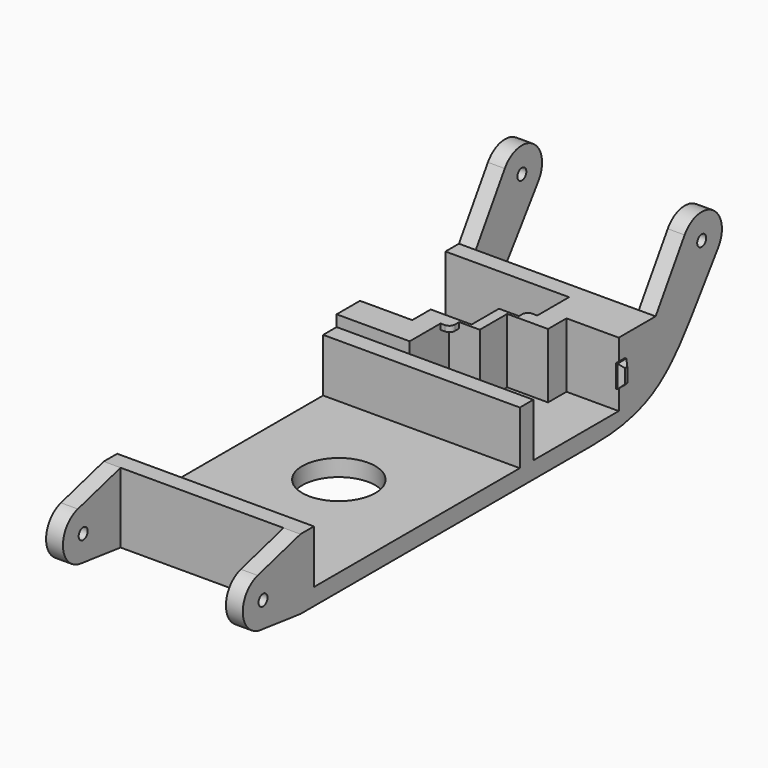
from build123d import *

# Parameters (mm, degrees)
F0_R      = 6.5
F0_W      = 34.999999702
F0_H      = 3
F0_H_2    = 0.3
F1_DEPTH  = 3
F2_DEPTH  = 9.5
F3_DEPTH  = 11.5
F5_DEPTH  = 3
F7_DEPTH  = 3
F8_R      = 1
F9_DEPTH  = 35.000999702
F11_DEPTH = 1
F13_DEPTH = 1
F14_SIZE  = 0.75
F15_W     = 1.8819853365
F15_H     = 1.731043148
F15_W_2   = 1.7636035271
F15_H_2   = 1.938064149
F16_DEPTH = 1
F18_DEPTH = 36.000999702
F19_R     = 1


# Not quite as in the source:
# - ends of sketch curves that miss each other by under 0.0002 mm in the source are joined
# - a feature names something its author has since deleted; it is built from what else it names


with BuildPart() as f1:
    # F0 (on Top) → F1 (new body)
    with BuildSketch(Plane.XY):
        Polygon((7.8607099131, 16.1003852367), (-9.6392899379, 16.1003852367), (-9.6392899379, -29.3996147633), (25.3607097641, -29.3996147633), (25.3607097641, 16.1003852367), align=None)
        with Locations((7.8607099131, -2.2867515218)):
            Circle(F0_R, mode=Mode.SUBTRACT)
        with Locations((7.8607099131, -31.1996147633)):
            Rectangle(F0_W, F0_H)
        Polygon((-9.6392899379, 19.1003852367), (-9.6392899379, 16.1003852367), (7.8607099131, 16.1003852367), (25.3607097641, 16.1003852367), (25.3607097641, 19.1003852367), (22.192974557, 19.1003852367), (3.3607097641, 19.1003852367), align=None)
        Polygon((-9.6392899379, 46.3003852367), (-9.6392899379, 43.3003852367), (-6.4715547308, 43.3003852367), (12.3607100621, 43.3003852367), (25.3607097641, 43.3003852367), (25.3607097641, 46.3003852367), align=None)
        with Locations((7.8607099131, -29.5496147633)):
            Rectangle(F0_W, F0_H_2)
        Polygon((16.0607097641, 38.1003852367), (25.3607097641, 38.1003852367), (25.3607097641, 43.3003852367), (12.3607100621, 43.3003852367), (12.3607100621, 35.3003852367), (12.3607100621, 34.5003852367), (7.8607097641, 34.5003852367), (7.8607100621, 33.9926332235), (8.7954637781, 33.9926332235), (16.0607097641, 33.9926332235), align=None)
        Polygon((-9.6392899379, 24.3003852367), (-9.6392899379, 19.1003852367), (3.3607097641, 19.1003852367), (3.3607097641, 27.1003852367), (3.3607097641, 27.9003852367), (7.8607100621, 27.9003852367), (7.8607100621, 28.4081372499), (6.9259563461, 28.4081372499), (-0.3392899379, 28.4081372499), (-0.3392899379, 24.3003852367), align=None)
        Polygon((6.9259563461, 34.5003852367), (6.9259563461, 28.4081372499), (7.8607097641, 28.4081372499), (7.8607100621, 33.9926332235), (7.8607100621, 34.5003852367), align=None)
        Polygon((7.8607100621, 28.4081372499), (7.8607100621, 27.9003852367), (8.7954637781, 27.9003852367), (8.7954637781, 33.9926332235), (7.8607097641, 33.9926332235), align=None)
        Polygon((-9.6392899379, 43.3003852367), (-9.6392899379, 24.3003852367), (-0.3392899379, 24.3003852367), (-0.3392899379, 28.4081372499), (6.9259563461, 28.4081372499), (6.9259563461, 34.5003852367), (7.8607100621, 34.5003852367), (12.3607100621, 34.5003852367), (12.3607100621, 35.3003852367), (12.3607100621, 43.3003852367), (-6.4715547308, 43.3003852367), align=None)
        Polygon((3.3607097641, 27.1003852367), (3.3607097641, 19.1003852367), (22.192974557, 19.1003852367), (25.3607097641, 19.1003852367), (25.3607097641, 38.1003852367), (16.0607097641, 38.1003852367), (16.0607097641, 33.9926332235), (8.7954637781, 33.9926332235), (8.7954637781, 27.9003852367), (7.8607100621, 27.9003852367), (3.3607097641, 27.9003852367), align=None)
    extrude(amount=-F1_DEPTH)

    # F0 (on Top) → F2 (join)
    with BuildSketch(Plane.XY):
        with Locations((7.8607099131, -31.1996147633)):
            Rectangle(F0_W, F0_H)
        Polygon((-9.6392899379, 19.1003852367), (-9.6392899379, 16.1003852367), (7.8607099131, 16.1003852367), (25.3607097641, 16.1003852367), (25.3607097641, 19.1003852367), (22.192974557, 19.1003852367), (3.3607097641, 19.1003852367), align=None)
    extrude(amount=F2_DEPTH)

    # F0 (on Top) → F3 (join)
    with BuildSketch(Plane.XY):
        Polygon((-9.6392899379, 46.3003852367), (-9.6392899379, 43.3003852367), (-6.4715547308, 43.3003852367), (12.3607100621, 43.3003852367), (25.3607097641, 43.3003852367), (25.3607097641, 46.3003852367), align=None)
        Polygon((-9.6392899379, 24.3003852367), (-9.6392899379, 19.1003852367), (3.3607097641, 19.1003852367), (3.3607097641, 27.1003852367), (3.3607097641, 27.9003852367), (7.8607100621, 27.9003852367), (7.8607100621, 28.4081372499), (6.9259563461, 28.4081372499), (-0.3392899379, 28.4081372499), (-0.3392899379, 24.3003852367), align=None)
        Polygon((7.8607100621, 28.4081372499), (7.8607100621, 27.9003852367), (8.7954637781, 27.9003852367), (8.7954637781, 33.9926332235), (7.8607097641, 33.9926332235), align=None)
        Polygon((6.9259563461, 34.5003852367), (6.9259563461, 28.4081372499), (7.8607097641, 28.4081372499), (7.8607100621, 33.9926332235), (7.8607100621, 34.5003852367), align=None)
        Polygon((16.0607097641, 38.1003852367), (25.3607097641, 38.1003852367), (25.3607097641, 43.3003852367), (12.3607100621, 43.3003852367), (12.3607100621, 35.3003852367), (12.3607100621, 34.5003852367), (7.8607097641, 34.5003852367), (7.8607100621, 33.9926332235), (8.7954637781, 33.9926332235), (16.0607097641, 33.9926332235), align=None)
    extrude(amount=F3_DEPTH)

    # F4 (on face) → F5 (join)
    with BuildSketch(Plane.YZ.offset(25.3607097641)):
        Polygon((-32.6996147633, -3), (46.3003852367, -3), (46.3003852367, 11.5), (38.1003852367, 11.5), (38.1003852367, 0), (19.1003852367, 0), (19.1003852367, 9.5), (16.1003852367, 9.5), (16.1003852367, 0), (-29.6996147633, 0), (-29.6996147633, 9.5), (-32.6996147633, 9.5), align=None)
        with BuildLine():
            Line((46.3003852367, 11.5), (46.3003852367, -3))
            Line((46.3003852367, -3), (60.2135883006, 16.6053474951))
            ThreePointArc((60.2135883006, 16.6053474951), (54.0324103863, 15.4756413664), (52.7478740756, 21.6265082006))
            Line((52.7478740756, 21.6265082006), (46.3003852367, 11.5))
        make_face()
        with BuildLine():
            ThreePointArc((52.7478740756, 21.6265082006), (54.0324103863, 15.4756413664), (60.2135883006, 16.6053474951))
            ThreePointArc((60.2135883006, 16.6053474951), (60.8312132136, 17.8429507129), (61.0437823534, 19.2096754909))
            ThreePointArc((61.0437823534, 19.2096754909), (57.8024349564, 23.5300682537), (52.7478740756, 21.6265082006))
        make_face()
        with BuildLine():
            Line((-41.5630528886, -1.9133363436), (-32.6996147633, -3))
            Line((-32.6996147633, -3), (-32.6996147633, 9.5))
            Line((-32.6996147633, 9.5), (-42.2056278, 6.8929759665))
            ThreePointArc((-42.2056278, 6.8929759665), (-38.2865124349, 6.1313346687), (-36.5154499114, 2.5532206055))
            ThreePointArc((-36.5154499114, 2.5532206055), (-38.0333544566, -0.8168100619), (-41.5630528886, -1.9133363436))
        make_face()
        with BuildLine():
            ThreePointArc((-42.2056278, 6.8929759665), (-45.503517949, 2.2257373389), (-41.5630528886, -1.9133363436))
            ThreePointArc((-41.5630528886, -1.9133363436), (-38.0333544566, -0.8168100619), (-36.5154499114, 2.5532206055))
            ThreePointArc((-36.5154499114, 2.5532206055), (-38.2865124349, 6.1313346687), (-42.2056278, 6.8929759665))
        make_face()
    extrude(amount=-F5_DEPTH)

    # F6 (on face) → F7 (join)
    with BuildSketch(Plane(origin=(-9.6392899379, 0, 0), x_dir=(0, -1, 0), z_dir=(-1, 0, 0))):
        with BuildLine():
            Line((-60.2135883006, 16.6053474951), (-46.3003852367, -3))
            Line((-46.3003852367, -3), (-46.3003852367, 11.5))
            Line((-46.3003852367, 11.5), (-52.7478740756, 21.6265082006))
            ThreePointArc((-52.7478740756, 21.6265082006), (-59.0551543205, 22.9437096154), (-60.2135883006, 16.6053474951))
        make_face()
        Polygon((-46.3003852367, 11.5), (-46.3003852367, -3), (32.6996147633, -3), (32.6996147633, 9.5), (29.6996147633, 9.5), (29.6996147633, 0), (-16.1003852367, 0), (-16.1003852367, 9.5), (-19.1003852367, 9.5), (-19.1003852367, 11.5), (-24.3003852367, 11.5), (-24.3003852367, 0), (-43.3003852367, 0), (-43.3003852367, 11.5), align=None)
        with BuildLine():
            Line((32.6996147633, 9.5), (32.6996147633, -3))
            Line((32.6996147633, -3), (41.5630528886, -1.9133363436))
            ThreePointArc((41.5630528886, -1.9133363436), (45.503517949, 2.2257373389), (42.2056278, 6.8929759665))
            Line((42.2056278, 6.8929759665), (32.6996147633, 9.5))
        make_face()
    extrude(amount=-F7_DEPTH)

    # F8 (on face) → F9 (cut, through all)
    with BuildSketch(Plane(origin=(-9.6392899379, 0, 0), x_dir=(0, -1, 0), z_dir=(-1, 0, 0))):
        with Locations((-56.5437823534, 19.2096754909)):
            Circle(F8_R)
        with Locations((41.0154499114, 2.5532206055)):
            Circle(F8_R)
    extrude(amount=-F9_DEPTH, mode=Mode.SUBTRACT)

    # F10 (on face) → F11 (join)
    with BuildSketch(Plane.YZ.offset(25.3607097641)):
        Polygon((39.4906885922, 7.75), (38.1003852367, 7.75), (38.1003852367, 3.75), (39.4906885922, 3.75), (39.4906885922, 5.75), align=None)
        Polygon((38.1003852367, 3.75), (38.1003852367, 7.75), (37.4906885922, 7.75), (37.4906885922, 5.75), (37.4906885922, 3.75), align=None)
    extrude(amount=F11_DEPTH)

    # F12 (on face) → F13 (join)
    with BuildSketch(Plane(origin=(-9.6392899379, 0, 0), x_dir=(0, -1, 0), z_dir=(-1, 0, 0))):
        Polygon((-22.9083076119, 7.75), (-24.3003852367, 7.75), (-24.3003852367, 3.75), (-22.9083076119, 3.75), (-22.9083076119, 5.75), align=None)
        Polygon((-24.9083076119, 7.75), (-24.9083076119, 5.75), (-24.9083076119, 3.75), (-24.3003852367, 3.75), (-24.3003852367, 7.75), align=None)
    extrude(amount=F13_DEPTH)

    # F14
    f14_edges = [f1.edges().sort_by_distance(p)[0] for p in [
        (-10.63929, 24.908308, 5.75),
        (-10.63929, 22.908308, 5.75),
        (-10.63929, 23.908308, 7.75),
        (-10.63929, 23.908308, 3.75),
        (26.36071, 38.490689, 7.75),
        (26.36071, 37.490689, 5.75),
        (26.36071, 38.490689, 3.75),
        (26.36071, 39.490689, 5.75),
    ]]
    chamfer(f14_edges, length=F14_SIZE)

    # F15 (on face) → F16 (join)
    with BuildSketch(Plane.XY.offset(11.5)):
        with Locations((11.4197173938, 35.3659068108)):
            Rectangle(F15_W, F15_H)
        with Locations((4.2425115276, 26.9313531622)):
            Rectangle(F15_W_2, F15_H_2)
    extrude(amount=-F16_DEPTH)

    # F17 (on face) → F18 (cut, through all)
    with BuildSketch(Plane(origin=(-9.6392899379, 0, 0), x_dir=(0, -1, 0), z_dir=(-1, 0, 0))):
        with BuildLine():
            Line((-56.1974216606, 10.9460940352), (-46.3003852367, -3))
            Line((-46.3003852367, -3), (-32.2360508144, -3))
            add(Edge.make_bspline(
                [(-56.1974216606, 10.9460940352), (-49.7821666885, 1.9062415714), (-46.3003852367, -3), (-32.2360508144, -3)],
                knots=[0, 0, 0, 0, 27.7243725207, 27.7243725207, 27.7243725207, 27.7243725207], degree=3))
        make_face()
    extrude(amount=-F18_DEPTH, mode=Mode.SUBTRACT)

    # F19
    f19_edges = [f1.edges().sort_by_distance(p)[0] for p in [
        (5.124313, 25.962321, 11),
        (10.478725, 36.231428, 11),
    ]]
    fillet(f19_edges, radius=F19_R)


solid = f1.part
